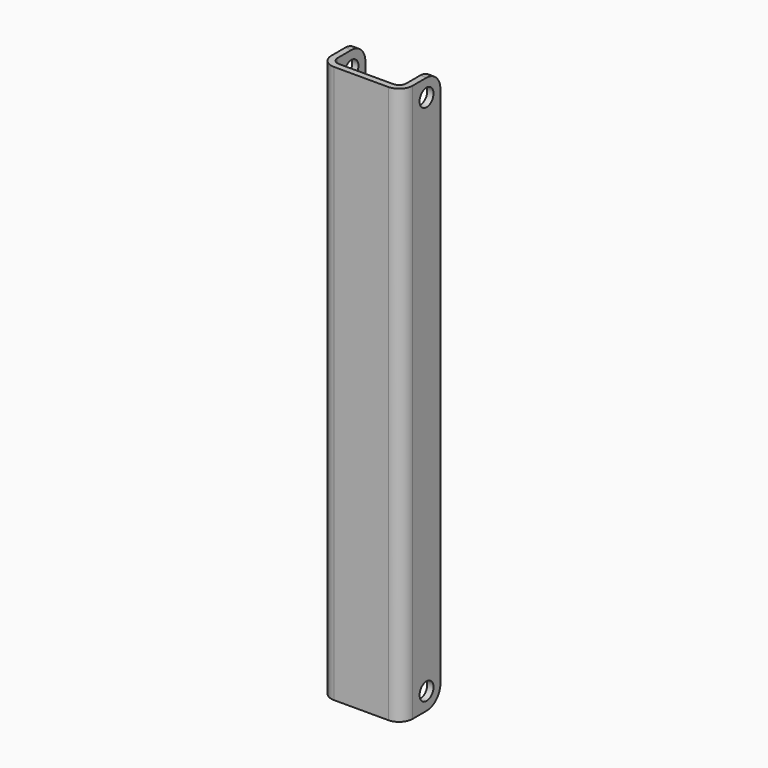
from build123d import *

# Parameters (mm, degrees)
F1_DEPTH = 152.4
F2_R     = 1.98374
F3_R     = 3.69316
F4_R     = 4.7625
F5_R     = 2.38125
F6_DEPTH = 22.225


with BuildPart() as f1:
    # F0 (on Top) → F1 (new body)
    with BuildSketch(Plane.XY):
        Polygon((0, 11.50874), (0, 0), (-18.80616, 0), (-18.80616, 11.50874), (-20.51558, 11.50874), (-20.51558, -1.70942), (1.70942, -1.70942), (1.70942, 11.50874), align=None)
    extrude(amount=F1_DEPTH)

    # F2
    f2_edges = [f1.edges().sort_by_distance(p)[0] for p in [
        (0, 0, 76.2),
        (-18.80616, 0, 76.2),
    ]]
    fillet(f2_edges, radius=F2_R)

    # F3
    f3_edges = [f1.edges().sort_by_distance(p)[0] for p in [
        (1.70942, -1.70942, 76.2),
        (-20.51558, -1.70942, 76.2),
    ]]
    fillet(f3_edges, radius=F3_R)

    # F4
    f4_edges = [f1.edges().sort_by_distance(p)[0] for p in [
        (0.85471, 11.50874, 152.4),
        (-19.66087, 11.50874, 152.4),
        (-19.66087, 11.50874, 0),
        (0.85471, 11.50874, 0),
    ]]
    fillet(f4_edges, radius=F4_R)

    # F5 (on face) → F6 (cut, through all)
    with BuildSketch(Plane.YZ.offset(1.70942)):
        with Locations((6.74624, 4.7625)):
            Circle(F5_R)
        with Locations((6.74624, 147.6375)):
            Circle(F5_R)
    extrude(amount=-F6_DEPTH, mode=Mode.SUBTRACT)


solid = f1.part
